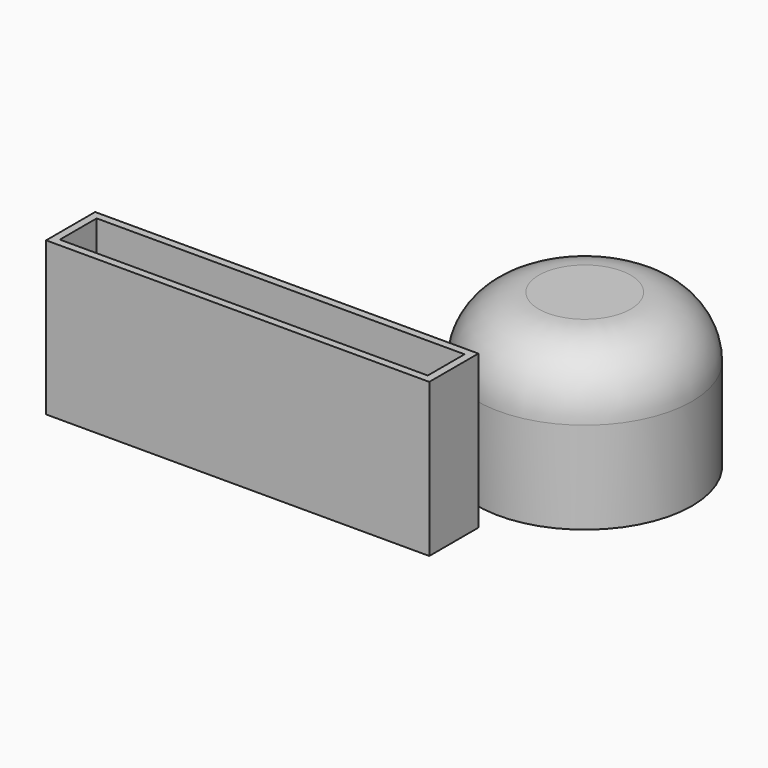
from build123d import *

# Parameters (mm, degrees)
F0_W     = 125
F0_H     = 20
F1_DEPTH = 50
F0_R     = 35
F2_R     = 20
F3_T     = -2.5


with BuildPart() as f1:
    # F0 (on Top) → F1 (new body)
    with BuildSketch(Plane.XY):
        with Locations((-62.5, 10)):
            Rectangle(F0_W, F0_H)
    extrude(amount=F1_DEPTH)

    # F3
    f3_openings = [f1.faces().sort_by_distance(p)[0] for p in [
        (-62.5, 10, 50),
    ]]
    offset(amount=F3_T, openings=f3_openings)


with BuildPart() as f1b:
    # F0 (on Top) → F1, piece 2 (new body)
    with BuildSketch(Plane.XY):
        with Locations((0, 63.3805897062)):
            Circle(F0_R)
    extrude(amount=F1_DEPTH)

    # F2
    f2_edges = [f1b.edges().sort_by_distance(p)[0] for p in [
        (-35, 63.38059, 50),
    ]]
    fillet(f2_edges, radius=F2_R)


solid = Compound([f1.part, f1b.part])
